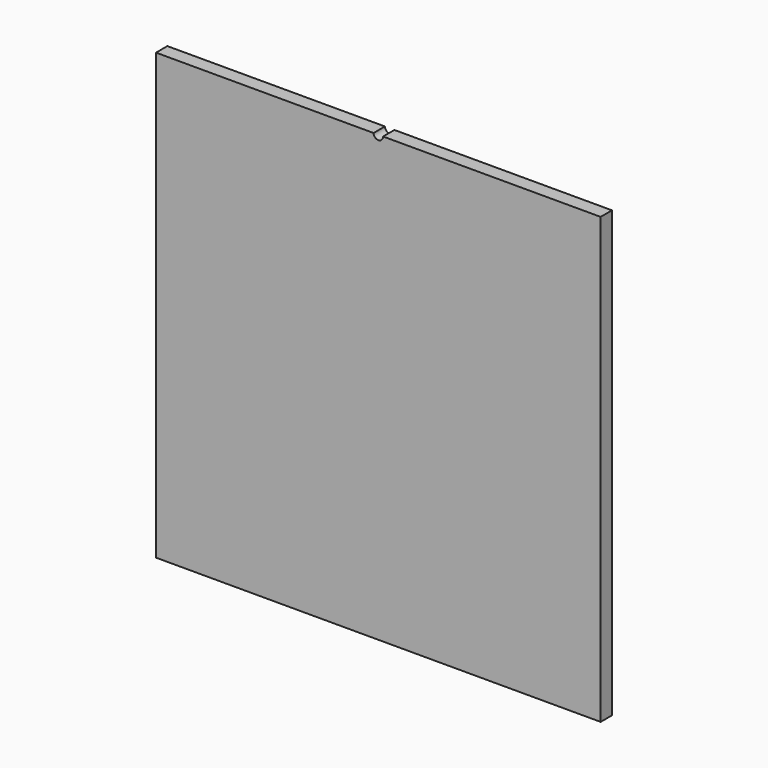
from build123d import *

# Parameters (mm, degrees)
F0_W     = 94
F0_H     = 94
F1_DEPTH = 3
F2_W     = 45
F2_H     = 15
F3_DEPTH = 3
F4_R     = 2.5796875
F5_DEPTH = 3.001
F6_R     = 5.159375
F7_DEPTH = 1.5875
F8_R     = 1
F9_DEPTH = 18.001


# Not quite as in the source:
# - a length typed as a fraction of an inch, garbled in the dataset ("3 / 203.2 mm" for 3/8 in), is restored


with BuildPart() as f1:
    # F0 (on Front) → F1 (new body)
    with BuildSketch(Plane.XZ):
        Rectangle(F0_W, F0_H)
    extrude(amount=F1_DEPTH)

    # F2 (on face) → F3 (join)
    with BuildSketch(Plane(origin=(0, 0, -47), x_dir=(1, 0, 0), z_dir=(0, 0, -1))):
        with Locations((0, -7.5)):
            Rectangle(F2_W, F2_H)
    extrude(amount=-F3_DEPTH)

    # F4 (on face) → F5 (cut, through all)
    with BuildSketch(Plane.XY.offset(-44)):
        with Locations((-15, 6)):
            Circle(F4_R)
        with Locations((15, 6)):
            Circle(F4_R)
    extrude(amount=-F5_DEPTH, mode=Mode.SUBTRACT)

    # F6 (on face) → F7 (cut)
    with BuildSketch(Plane.XY.offset(-44)):
        with Locations((-15, 6)):
            Circle(F6_R)
        with Locations((15, 6)):
            Circle(F6_R)
    extrude(amount=-F7_DEPTH, mode=Mode.SUBTRACT)

    # F8 (on face) → F9 (cut, through all)
    with BuildSketch(Plane.XZ.offset(3)):
        with Locations((0, 47)):
            Circle(F8_R)
    extrude(amount=-F9_DEPTH, mode=Mode.SUBTRACT)


solid = f1.part
